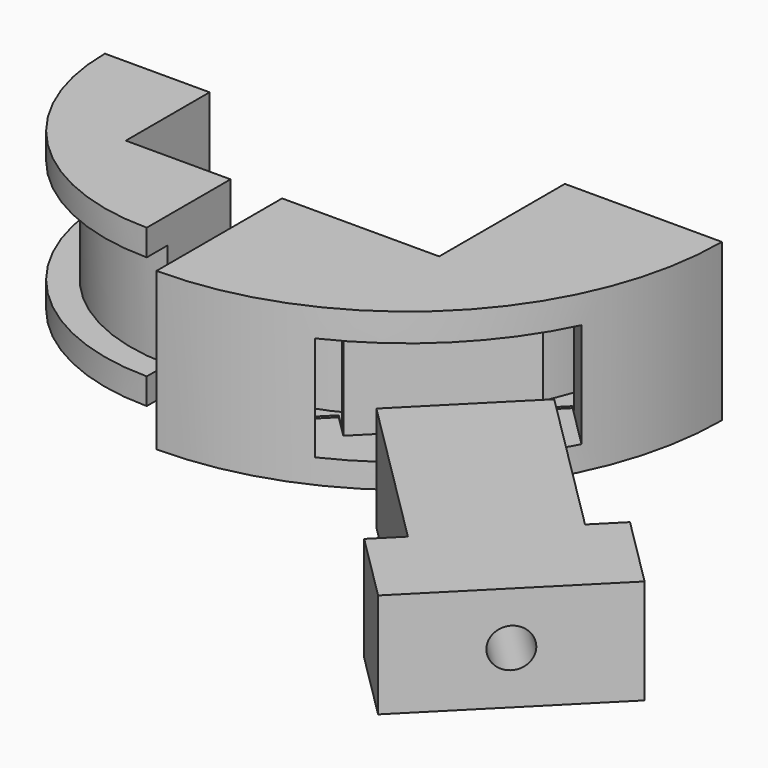
from build123d import *

# Parameters (mm, degrees)
F1_DEPTH  = 38.1
F2_W      = 6.35
F2_H      = 25.4
F3_ANGLE  = 91
F5_DEPTH  = 38.1
F6_W      = 6.35
F6_H      = 25.4
F7_ANGLE  = 30
F11_W     = 50.8
F11_H     = 25.4
F12_DEPTH = 38.1
F8_W      = 6.35
F8_H      = 25.4
F13_ANGLE = 30
F14_W     = 6.35
F14_H     = 25.4
F15_DEPTH = 7.62
F16_W     = 6.35
F16_H     = 25.4
F17_DEPTH = 6.35
F18_DEPTH = 76.2
F19_R     = 4.7625
F20_DEPTH = 76.2
F22_DEPTH = 25.4


# Not quite as in the source:
# - a feature names something its author has since deleted; it is built from what else it names


with BuildPart() as f1:
    # F0 (on Top) → F1 (new body)
    with BuildSketch(Plane.XY):
        with BuildLine():
            Line((0, 25.4), (-25.4, 25.4))
            ThreePointArc((-25.4, 25.4), (-10.5210244843, -10.5210244843), (25.4, -25.4))
            Line((25.4, -25.4), (25.4, 0))
            Line((25.4, 0), (0, 0))
            Line((0, 0), (0, 25.4))
        make_face()
    extrude(amount=F1_DEPTH)

    # F2 (on face) → F3 (revolve, cut)
    with BuildSketch(Plane.YZ.offset(25.4)):
        with Locations((-28.575, 19.05)):
            Rectangle(F2_W, F2_H)
        with Locations((-22.225, 19.05)):
            Rectangle(F2_W, F2_H)
    revolve(axis=Axis((25.4, 25.3727845848, 25.4265852273), (0, 0, -1)), revolution_arc=F3_ANGLE, mode=Mode.SUBTRACT)


with BuildPart() as f5:
    # F4 (on Top) → F5 (new body)
    with BuildSketch(Plane.XY):
        with BuildLine():
            Line((114.1095044971, 38.1), (76.0095044971, 38.1))
            Line((76.0095044971, 38.1), (76.0095044971, 0))
            Line((76.0095044971, 0), (37.9095044971, 0))
            Line((37.9095044971, 0), (37.9095044971, -38.1))
            ThreePointArc((37.9095044971, -38.1), (91.7910412235, -15.7815367264), (114.1095044971, 38.1))
        make_face()
    extrude(amount=F5_DEPTH)

    # F6 (on face) → F7 (revolve, cut)
    with BuildSketch(Plane(origin=(37.9095044971, 0, 0), x_dir=(0, -1, 0), z_dir=(-1, 0, 0))):
        with Locations((22.86, 19.05)):
            Rectangle(F6_W, F6_H)
    revolve(axis=Axis((37.9095044971, 38.3080989122, 33.1992767751), (0, 0, 1)), revolution_arc=F7_ANGLE, mode=Mode.SUBTRACT)

    # F11 (on face) → F12 (cut)
    with BuildSketch(Plane(origin=(72.0218737811, -71.6617729132, 0), x_dir=(0.7053324106, 0.7088767104, 0), z_dir=(0.7088767104, -0.7053324106, 0))):
        with Locations((53.2859638333, 18.6154339463)):
            Rectangle(F11_W, F11_H)
    extrude(amount=-F12_DEPTH, mode=Mode.SUBTRACT)

    # F8 (on face) → F13 (revolve, cut)
    with BuildSketch(Plane(origin=(0, 38.1, 0), x_dir=(-1, 0, 0), z_dir=(0, 1, 0))):
        with Locations((-98.8695044971, 19.05)):
            Rectangle(F8_W, F8_H)
    revolve(axis=Axis((38.0943529308, 38.1, 28.2714888453), (0, 0, -1)), revolution_arc=F13_ANGLE, mode=Mode.SUBTRACT)

    # F14 (on face) → F15 (cut)
    with BuildSketch(Plane(origin=(45.0136711132, -44.7886080707, 0), x_dir=(0.7053324106, 0.7088767104, 0), z_dir=(0.7088767104, -0.7053324106, 0))):
        with Locations((31.0609638333, 18.6154339463)):
            Rectangle(F14_W, F14_H)
    extrude(amount=-F15_DEPTH, mode=Mode.SUBTRACT)

    # F16 (on face) → F17 (cut)
    with BuildSketch(Plane(origin=(45.0136711132, -44.7886080707, 0), x_dir=(0.7053324106, 0.7088767104, 0), z_dir=(0.7088767104, -0.7053324106, 0))):
        with Locations((75.5109638333, 18.6154339463)):
            Rectangle(F16_W, F16_H)
    extrude(amount=-F17_DEPTH, mode=Mode.SUBTRACT)


with BuildPart() as f18:
    # F11 (on face) → F18 (new body)
    with BuildSketch(Plane(origin=(72.0218737811, -71.6617729132, 0), x_dir=(0.7053324106, 0.7088767104, 0), z_dir=(0.7088767104, -0.7053324106, 0))):
        with Locations((53.2859638333, 18.6154339463)):
            Rectangle(F11_W, F11_H)
    extrude(amount=F18_DEPTH)

    # F19 (on face) → F20 (cut)
    with BuildSketch(Plane(origin=(126.038279117, -125.408102598, 0), x_dir=(0.7053324106, 0.7088767104, 0), z_dir=(0.7088767104, -0.7053324106, 0))):
        with Locations((53.2859638333, 18.6154339463)):
            Circle(F19_R)
    extrude(amount=-F20_DEPTH, mode=Mode.SUBTRACT)

    # F21 (on face) → F22 (cut)
    with BuildSketch(Plane.XY.offset(31.3154339463)):
        Polygon((135.04124021, -83.2723715078), (97.5683920804, -45.9868831958), (91.6907478725, -51.8940626034), (129.1635960022, -89.1795509154), align=None)
        Polygon((127.5216343291, -15.8831257129), (121.4778258094, -21.9573044091), (158.1326163355, -58.428825309), (164.1764248552, -52.3546466128), align=None)
    extrude(amount=-F22_DEPTH, mode=Mode.SUBTRACT)


solid = Compound([f1.part, f5.part, f18.part])
